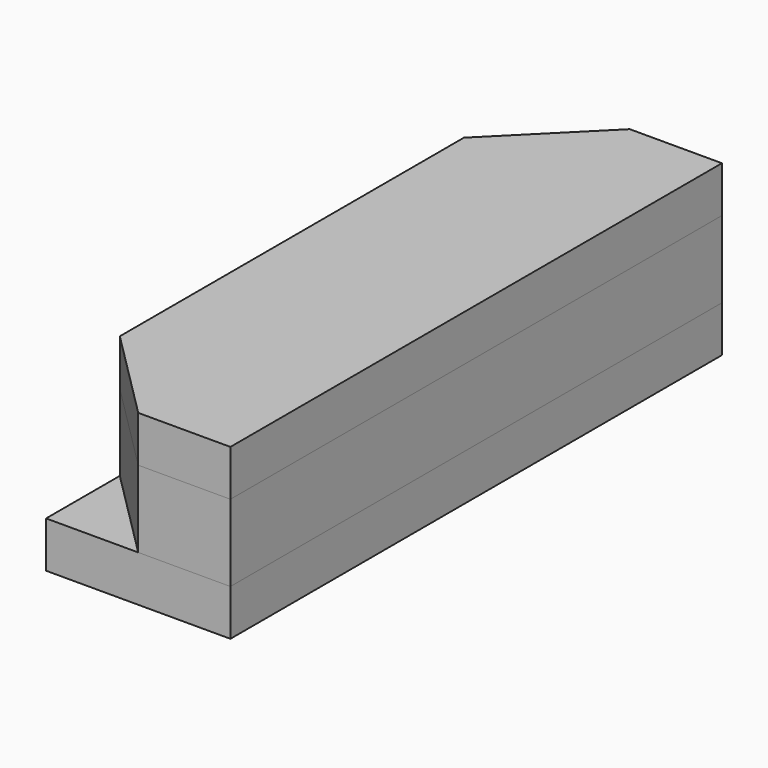
from build123d import *

# Parameters (mm, degrees)
F1_DEPTH  = 4
F3_W      = 6
F3_H      = 20
F4_DEPTH  = 1.5
F5_SIZE   = 3
F5_2_SIZE = 3


with BuildPart() as f1:
    # F0 (on Top) → F1 (new body)
    with BuildSketch(Plane.XY):
        with BuildLine():
            Line((3, -10), (3, 10))
            Line((3, 10), (-3, 10))
            Line((-3, 10), (-3, 5.8113613003))
            ThreePointArc((-3, 5.8113613003), (0.5654981212, 4.3166748595), (1.9992755637, 0.7262505595))
            Line((1.9992755637, 0.7262505595), (1.9999993434, -0.6860763339))
            ThreePointArc((1.9999993434, -0.6860763339), (0.536439723, -4.2232665564), (-3, -5.6886386997))
            Line((-3, -5.6886386997), (-3, -10))
            Line((-3, -10), (3, -10))
        make_face()
    extrude(amount=F1_DEPTH)

    # F5
    f5_edges = [f1.edges().sort_by_distance(p)[0] for p in [
        (-3, 10, 2),
        (-3, -10, 2),
    ]]
    chamfer(f5_edges, length=F5_SIZE)


with BuildPart() as f1b:
    # F0 (on Top) → F1, piece 2 (new body)
    with BuildSketch(Plane.XY):
        with BuildLine():
            ThreePointArc((-3, 2.3113613003), (-1.9227647543, 1.8551832321), (-1.5007442997, 0.7641136008))
            Line((-1.5007442997, 0.7641136008), (-1.500000197, -0.68786999))
            ThreePointArc((-1.500000197, -0.68786999), (-1.9390680831, -1.7490270567), (-3, -2.1886386997))
            Line((-3, -2.1886386997), (-3, -3.9386386997))
            ThreePointArc((-3, -3.9386386997), (-0.70131418, -2.9861468066), (0.2499995732, -0.6869731619))
            Line((0.2499995732, -0.6869731619), (0.2492670865, 0.7423439064))
            ThreePointArc((0.2492670865, 0.7423439064), (-0.6776298174, 3.084926064), (-3, 4.0613613003))
            Line((-3, 4.0613613003), (-3, 2.3113613003))
        make_face()
    extrude(amount=F1_DEPTH)


with BuildPart() as f4:
    # F3 (on face) → F4 (new body)
    with BuildSketch(Plane.XY.offset(4)):
        Rectangle(F3_W, F3_H)
    extrude(amount=F4_DEPTH)

    # F5#2
    f5_2_edges = [f4.edges().sort_by_distance(p)[0] for p in [
        (-3, 10, 4.75),
        (-3, -10, 4.75),
    ]]
    chamfer(f5_2_edges, length=F5_2_SIZE)


with BuildPart() as f4b:
    # F0 (on Top) → F4, piece 2 (new body)
    with BuildSketch(Plane.XY):
        with BuildLine():
            Line((3, -10), (3, 10))
            Line((3, 10), (-3, 10))
            Line((-3, 10), (-3, 5.8113613003))
            ThreePointArc((-3, 5.8113613003), (0.5654981212, 4.3166748595), (1.9992755637, 0.7262505595))
            Line((1.9992755637, 0.7262505595), (1.9999993434, -0.6860763339))
            ThreePointArc((1.9999993434, -0.6860763339), (0.536439723, -4.2232665564), (-3, -5.6886386997))
            Line((-3, -5.6886386997), (-3, -10))
            Line((-3, -10), (3, -10))
        make_face()
    extrude(amount=F4_DEPTH)


with BuildPart() as f4c:
    # F0 (on Top) → F4, piece 3 (new body)
    with BuildSketch(Plane.XY):
        with BuildLine():
            ThreePointArc((-3, 2.3113613003), (-1.9227647543, 1.8551832321), (-1.5007442997, 0.7641136008))
            Line((-1.5007442997, 0.7641136008), (-1.500000197, -0.68786999))
            ThreePointArc((-1.500000197, -0.68786999), (-1.9390680831, -1.7490270567), (-3, -2.1886386997))
            Line((-3, -2.1886386997), (-3, -3.9386386997))
            ThreePointArc((-3, -3.9386386997), (-0.70131418, -2.9861468066), (0.2499995732, -0.6869731619))
            Line((0.2499995732, -0.6869731619), (0.2492670865, 0.7423439064))
            ThreePointArc((0.2492670865, 0.7423439064), (-0.6776298174, 3.084926064), (-3, 4.0613613003))
            Line((-3, 4.0613613003), (-3, 2.3113613003))
        make_face()
    extrude(amount=F4_DEPTH)


solid = Compound([f1.part, f1b.part, f4.part, f4b.part, f4c.part])
